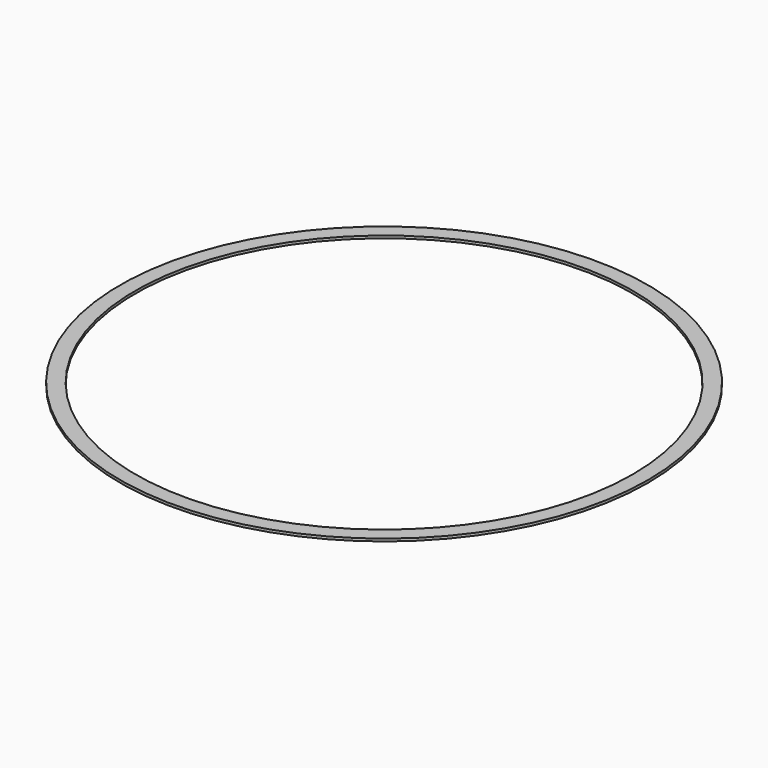
from build123d import *

# Parameters (mm, degrees)
F0_R     = 439.36285
F0_R_2   = 413.96285
F1_DEPTH = 4.2333333333


# Not quite as in the source:
# - a length typed as a fraction of an inch, garbled in the dataset ("3 / 203.2 mm" for 3/8 in), is restored


with BuildPart() as f1:
    # F0 (on Top) → F1 (new body)
    with BuildSketch(Plane.XY):
        Circle(F0_R)
        Circle(F0_R_2, mode=Mode.SUBTRACT)
    extrude(amount=F1_DEPTH)


solid = f1.part
